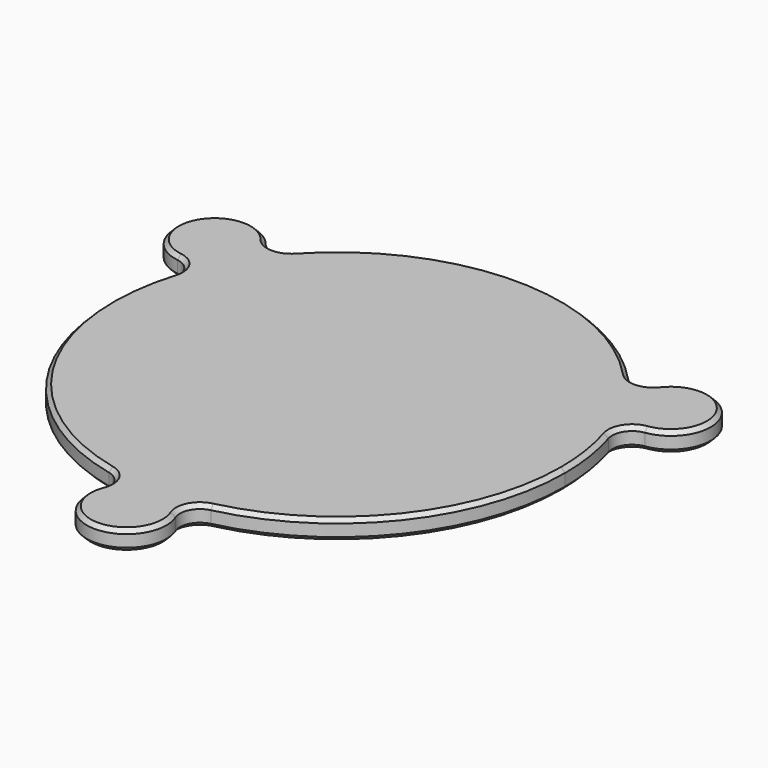
from build123d import *

# Parameters (mm, degrees)
F1_DEPTH = 5
F2_R     = 5
F3_SIZE  = 1


with BuildPart() as f1:
    # F0 (on Top) → F1 (new body)
    with BuildSketch(Plane.XY):
        with BuildLine():
            ThreePointArc((-4.0489926269, -57.0063869992), (0, -76.15), (4.0489926269, -57.0063869992))
            ThreePointArc((4.0489926269, -57.0063869992), (0, -57.15), (-4.0489926269, -57.0063869992))
        make_face()
        with BuildLine():
            ThreePointArc((4.0489926269, -57.0063869992), (41.8181923846, -38.9533218826), (57.15, 0))
            ThreePointArc((57.15, 0), (55.6922778867, 12.8254701198), (51.3934756327, 24.996663025))
            ThreePointArc((51.3934756327, 24.996663025), (49.4933518263, 28.575), (47.3444830059, 32.0097239742))
            ThreePointArc((47.3444830059, 32.0097239742), (0, 57.15), (-47.3444830059, 32.0097239742))
            ThreePointArc((-47.3444830059, 32.0097239742), (-49.4933518263, 28.575), (-51.3934756327, 24.996663025))
            ThreePointArc((-51.3934756327, 24.996663025), (-49.4933518263, -28.575), (-4.0489926269, -57.0063869992))
            ThreePointArc((-4.0489926269, -57.0063869992), (0, -57.15), (4.0489926269, -57.0063869992))
        make_face()
        with BuildLine():
            ThreePointArc((47.3444830059, 32.0097239742), (49.4933518263, 28.575), (51.3934756327, 24.996663025))
            ThreePointArc((51.3934756327, 24.996663025), (65.9478344982, 38.075), (47.3444830059, 32.0097239742))
        make_face()
        with BuildLine():
            ThreePointArc((-51.3934756327, 24.996663025), (-49.4933518263, 28.575), (-47.3444830059, 32.0097239742))
            ThreePointArc((-47.3444830059, 32.0097239742), (-65.9478344982, 38.075), (-51.3934756327, 24.996663025))
        make_face()
    extrude(amount=F1_DEPTH)

    # F2
    f2_edges = [f1.edges().sort_by_distance(p)[0] for p in [
        (-4.048993, -57.006387, 2.5),
        (51.393476, 24.996663, 2.5),
        (-47.344483, 32.009724, 2.5),
        (4.048993, -57.006387, 2.5),
        (47.344483, 32.009724, 2.5),
        (-51.393476, 24.996663, 2.5),
    ]]
    fillet(f2_edges, radius=F2_R)

    # F3
    f3_edges = [f1.edges().sort_by_distance(p)[0] for p in [
        (0, -76.15, 5),
        (-9.492901, -58.253155, 5),
        (9.492901, -58.253155, 5),
        (-49.493352, -28.575, 5),
        (49.493352, -28.575, 5),
        (-55.195163, 20.905484, 5),
        (55.195163, 20.905484, 5),
        (-65.947834, 38.075, 5),
        (65.947834, 38.075, 5),
        (-45.702262, 37.347671, 5),
        (45.702262, 37.347671, 5),
        (0, 57.15, 5),
        (0, -76.15, 0),
        (-9.492901, -58.253155, 0),
        (9.492901, -58.253155, 0),
        (-49.493352, -28.575, 0),
        (49.493352, -28.575, 0),
        (-55.195163, 20.905484, 0),
        (55.195163, 20.905484, 0),
        (-65.947834, 38.075, 0),
        (65.947834, 38.075, 0),
        (-45.702262, 37.347671, 0),
        (45.702262, 37.347671, 0),
        (0, 57.15, 0),
    ]]
    chamfer(f3_edges, length=F3_SIZE)


solid = f1.part
